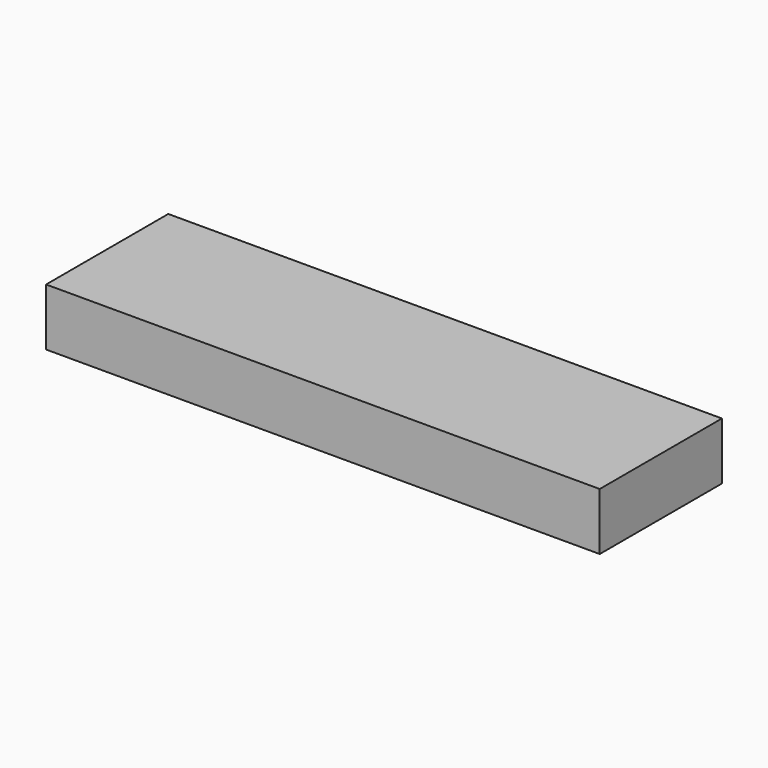
from build123d import *

# Parameters (mm, degrees)
F0_W     = 184.15
F0_H     = 50.8
F1_DEPTH = 19.05


# Not quite as in the source:
# - a length typed as a fraction of an inch, garbled in the dataset ("3 / 203.2 mm" for 3/8 in), is restored


with BuildPart() as f1:
    # F0 (on Top) → F1 (new body)
    with BuildSketch(Plane.XY):
        with Locations((-19.7819460869, 34.901772334)):
            Rectangle(F0_W, F0_H)
    extrude(amount=F1_DEPTH)


solid = f1.part
